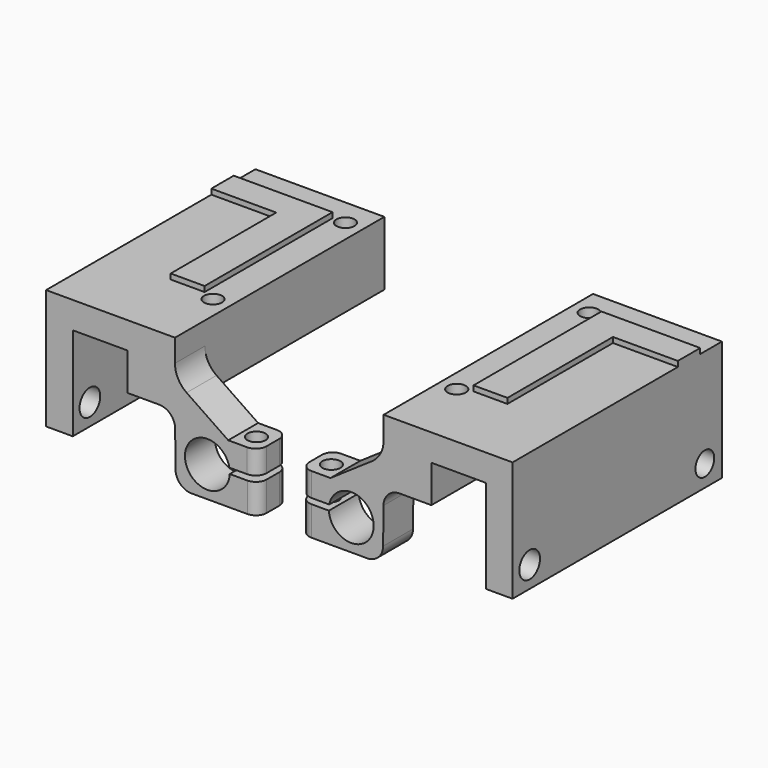
from build123d import *

# Parameters (mm, degrees)
F1_DEPTH      = 7
F2_DEPTH      = 42
F3_R          = 1.7
F3_R_2        = 11
F4_DEPTH      = 12.001
F5_R          = 4.2
F6_DEPTH      = 10
F7_DEPTH      = 12.001
F8_R          = 1.4
F9_DEPTH      = 10.9920075553
F8_R_2        = 1.7
F10_DEPTH     = 4.4348209087
F11_R         = 5
F12_R         = 3
F13_R         = 3
F14_R         = 2
F15_R         = 2.2
F15_R_2       = 2.4255023423
F16_DEPTH     = 6
F17_TEXT_SIZE = 41.9437823343
F18_DEPTH     = 1


# Not quite as in the source:
# - a feature names something its author has since deleted; it is built from what else it names
# - Text() gives the source's letters only with a copy of the font that has no kerning and outlines rounded to 1/6400 em; it was checked with that copy


with BuildPart() as f1:
    # F0 (on Front) → F1 (new body)
    with BuildSketch(Plane.XZ):
        Polygon((-18.6721007523, 29.8099789735), (-18.6721007523, 7.3259699669), (-13.6721007523, 7.3259699669), (-13.6721007523, 24.8099789735), (-3.4721007523, 24.8099789735), (-3.4721007523, 17.8099789735), (5.4637966118, 17.8099789735), (5.4637966118, 22.9406704692), (5.4637966118, 29.8099789735), align=None)
        Polygon((15.4301751077, 16.1394868046), (5.4637966118, 22.9406704692), (5.4637966118, 17.8099789735), (5.5940201178, 5.1484792493), (21.0186601057, 5.1484792493), (21.0186601057, 10.6682249423), (13.6860510706, 10.6682249423), (13.6860510706, 11.7046658959), (20.9896428882, 11.7046658959), (20.9896428882, 16.1394868046), align=None)
    extrude(amount=F1_DEPTH)

    # F0 (on Front) → F2 (join)
    with BuildSketch(Plane.XZ):
        Polygon((-18.6721007523, 29.8099789735), (-18.6721007523, 7.3259699669), (-13.6721007523, 7.3259699669), (-13.6721007523, 24.8099789735), (-3.4721007523, 24.8099789735), (-3.4721007523, 17.8099789735), (5.4637966118, 17.8099789735), (5.4637966118, 22.9406704692), (5.4637966118, 29.8099789735), align=None)
    extrude(amount=-F2_DEPTH)

    # F3 (on face) → F4 (cut, through all)
    with BuildSketch(Plane(origin=(0, 0, 17.8099789735), x_dir=(1, 0, 0), z_dir=(0, 0, -1))):
        with Locations((2.1850741468, -6)):
            Circle(F3_R)
        with Locations((2.1850741468, -37)):
            Circle(F3_R)
        with Locations((17.6850741468, -21.5)):
            Circle(F3_R_2)
    extrude(amount=-F4_DEPTH, mode=Mode.SUBTRACT)

    # F5 (on face) → F6 (cut)
    with BuildSketch(Plane.XZ.offset(7)):
        with Locations((11.5278992477, 10.8989789735)):
            Circle(F5_R)
    extrude(amount=-F6_DEPTH, mode=Mode.SUBTRACT)

    # F3 (on face) → F7 (cut, through all)
    with BuildSketch(Plane(origin=(0, 0, 17.8099789735), x_dir=(1, 0, 0), z_dir=(0, 0, -1))):
        with Locations((2.1850741468, -6)):
            Circle(F3_R)
        with Locations((2.1850741468, -37)):
            Circle(F3_R)
        with Locations((17.6850741468, -21.5)):
            Circle(F3_R_2)
    extrude(amount=-F7_DEPTH, mode=Mode.SUBTRACT)

    # F8 (on face) → F9 (cut, through all)
    with BuildSketch(Plane.XY.offset(16.1394868046)):
        with Locations((17.9896428882, -3.5767070949)):
            Circle(F8_R)
    extrude(amount=-F9_DEPTH, mode=Mode.SUBTRACT)

    # F8 (on face) → F10 (cut, through all)
    with BuildSketch(Plane.XY.offset(16.1394868046)):
        with Locations((17.9896428882, -3.5767070949)):
            Circle(F8_R_2)
        with Locations((17.9896428882, -3.5767070949)):
            Circle(F8_R, mode=Mode.SUBTRACT)
    extrude(amount=-F10_DEPTH, mode=Mode.SUBTRACT)

    # F11
    f11_edges = [f1.edges().sort_by_distance(p)[0] for p in [
        (5.463797, -3.5, 22.94067),
    ]]
    fillet(f11_edges, radius=F11_R)

    # F12
    f12_edges = [f1.edges().sort_by_distance(p)[0] for p in [
        (5.463797, -3.5, 17.809979),
    ]]
    fillet(f12_edges, radius=F12_R)

    # F13
    f13_edges = [f1.edges().sort_by_distance(p)[0] for p in [
        (5.59402, -3.5, 5.148479),
    ]]
    fillet(f13_edges, radius=F13_R)

    # F14
    f14_edges = [f1.edges().sort_by_distance(p)[0] for p in [
        (20.989643, -7, 13.922076),
        (21.01866, -7, 7.908352),
        (20.989643, 0, 13.922076),
        (21.01866, 0, 7.908352),
    ]]
    fillet(f14_edges, radius=F14_R)

    # F15 (on face) → F16 (cut)
    with BuildSketch(Plane(origin=(-18.6721007523, 0, 0), x_dir=(0, -1, 0), z_dir=(-1, 0, 0))):
        with Locations((-38, 11.3259699669)):
            Circle(F15_R)
        with Locations((3, 11.3259699669)):
            Circle(F15_R_2)
    extrude(amount=-F16_DEPTH, mode=Mode.SUBTRACT)

    # F17 (on face) → F18 (join)
    with BuildSketch(Plane.XY.offset(29.8099789735)):
        with Locations(Location((3.5908724648, 36.9253193088), (0, 0, 180))):
            Text('L', F17_TEXT_SIZE, font='Open Sans', font_style=FontStyle.BOLD, text_align=(TextAlign.LEFT, TextAlign.BOTTOM))
    extrude(amount=F18_DEPTH)


with BuildPart() as f19_1:
    # F19: instance of F1
    add(f1.part.mirror(Plane.YZ))


with BuildPart() as f19_1_1:
    # F20: moved
    add(f19_1.part.moved(Location((50, 0, 0))))


solid = Compound([f1.part, f19_1_1.part])
